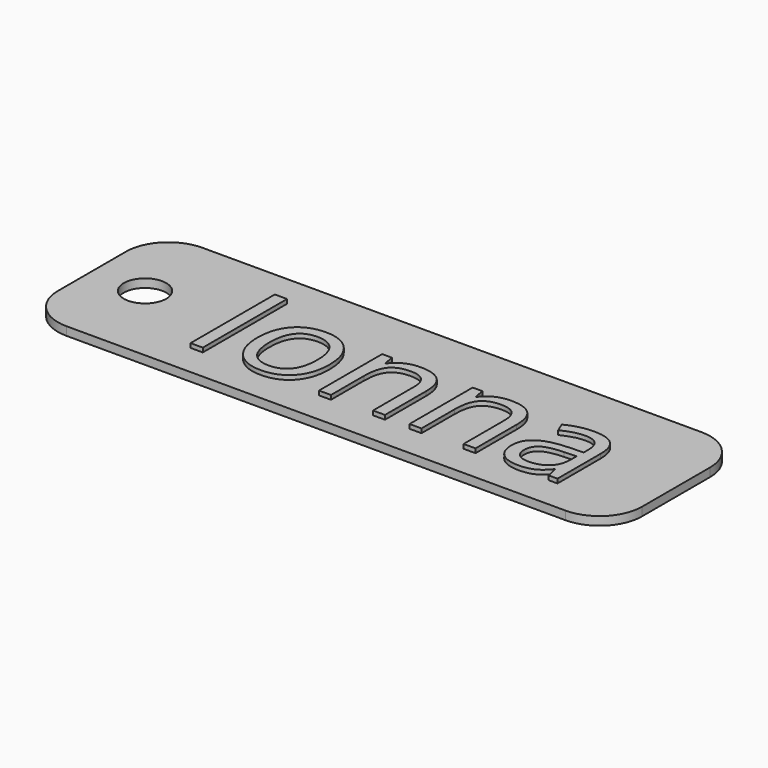
from build123d import *

# Parameters (mm, degrees)
F0_W         = 55
F0_H         = 16
F0_R         = 2
F1_DEPTH     = 0.8
F2_TEXT_SIZE = 13.8888888889
F3_DEPTH     = 0.4
F4_R         = 4


# Not quite as in the source:
# - Text() gives the source's letters only with a copy of the font that has no kerning and outlines rounded to 1/6400 em; it was checked with that copy


with BuildPart() as f1:
    # F0 (on Top) → F1 (new body)
    with BuildSketch(Plane.XY):
        Rectangle(F0_W, F0_H)
        with Locations((-22.5, 0)):
            Circle(F0_R, mode=Mode.SUBTRACT)
    extrude(amount=F1_DEPTH)

    # F2 (on face) → F3 (join)
    with BuildSketch(Plane.XY.offset(0.8)):
        with Locations((-15.5760282063, -5)):
            Text('Ionna', F2_TEXT_SIZE, font='Open Sans', text_align=(TextAlign.LEFT, TextAlign.BOTTOM))
    extrude(amount=F3_DEPTH)

    # F4
    f4_edges = [f1.edges().sort_by_distance(p)[0] for p in [
        (-27.5, -8, 0.4),
        (27.5, -8, 0.4),
        (27.5, 8, 0.4),
        (-27.5, 8, 0.4),
    ]]
    fillet(f4_edges, radius=F4_R)


solid = f1.part
